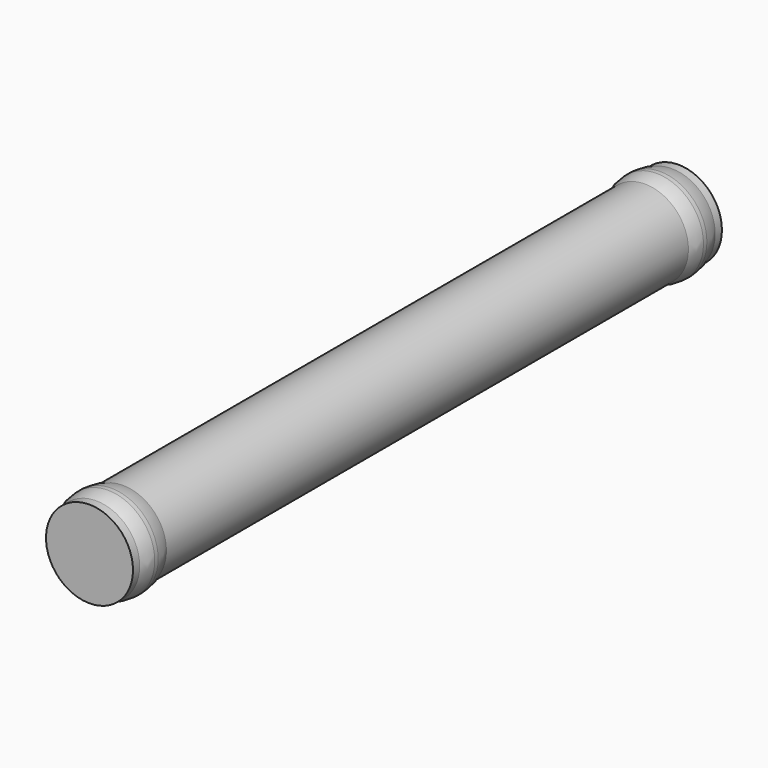
from build123d import *

# Parameters (mm, degrees)
F0_R     = 3.302
F1_DEPTH = 55.88
F3_R     = 3.556
F4_DEPTH = 1.27


# Not quite as in the source:
# - a fillet or chamfer that OpenCascade refuses, or shapes differently, is made with other operations: its cross-section is extruded or revolved along the edge and cut away or added
# - a feature names something its author has since deleted; it is built from what else it names


with BuildPart() as f1:
    # F0 (on Front) → F1 (new body)
    with BuildSketch(Plane.XZ):
        with Locations((-16.002, 0)):
            Circle(F0_R)
    extrude(amount=F1_DEPTH)

    # F3 (on offset) → F4 (join, symmetric)
    with BuildSketch(Plane.XZ.offset(53.975)):
        with Locations((-16.002, 0)):
            Circle(F3_R)
    extrude(amount=F4_DEPTH, both=True)

    # F6: F1 across plane


with BuildPart() as f1_1:
    add(f1.part)
    add(f1.part.mirror(Plane(origin=(-16.002, -27.94, 0), x_dir=(1, 0, 0), z_dir=(0, -1, 0))))

    # F7: fillet of radius 2.54 on 4 edges, made by hand

    # F7_s1 → F7_t2 (revolve, cut)
    with BuildSketch(Plane.XY):
        with BuildLine():
            ThreePointArc((-12.446, -54.1378396683), (-12.5103142364, -54.7058009346), (-12.7, -55.245))
            Line((-12.7, -55.245), (-12.446, -55.245))
            Line((-12.446, -55.245), (-12.446, -54.1378396683))
        make_face()
    revolve(axis=Axis((-16.002, -55.245, 0), (0, -1, 0)), mode=Mode.SUBTRACT)

    # F7_s3 → F7_t4 (revolve, cut)
    with BuildSketch(Plane.XY):
        with BuildLine():
            ThreePointArc((-12.7, -52.705), (-12.5103142364, -53.2441990654), (-12.446, -53.8121603317))
            Line((-12.446, -53.8121603317), (-12.446, -52.705))
            Line((-12.446, -52.705), (-12.7, -52.705))
        make_face()
    revolve(axis=Axis((-16.002, -52.705, 0), (0, -1, 0)), mode=Mode.SUBTRACT)

    # F7_s5 → F7_t6 (revolve, cut)
    with BuildSketch(Plane.XY):
        with BuildLine():
            ThreePointArc((-12.446, -2.0678396683), (-12.5103142364, -2.6358009346), (-12.7, -3.175))
            Line((-12.7, -3.175), (-12.446, -3.175))
            Line((-12.446, -3.175), (-12.446, -2.0678396683))
        make_face()
    revolve(axis=Axis((-16.002, -3.175, 0), (0, -1, 0)), mode=Mode.SUBTRACT)

    # F7_s7 → F7_t8 (revolve, cut)
    with BuildSketch(Plane.XY):
        with BuildLine():
            ThreePointArc((-12.7, -0.635), (-12.5103142364, -1.1741990654), (-12.446, -1.7421603317))
            Line((-12.446, -1.7421603317), (-12.446, -0.635))
            Line((-12.446, -0.635), (-12.7, -0.635))
        make_face()
    revolve(axis=Axis((-16.002, -0.635, 0), (0, -1, 0)), mode=Mode.SUBTRACT)


solid = f1_1.part
